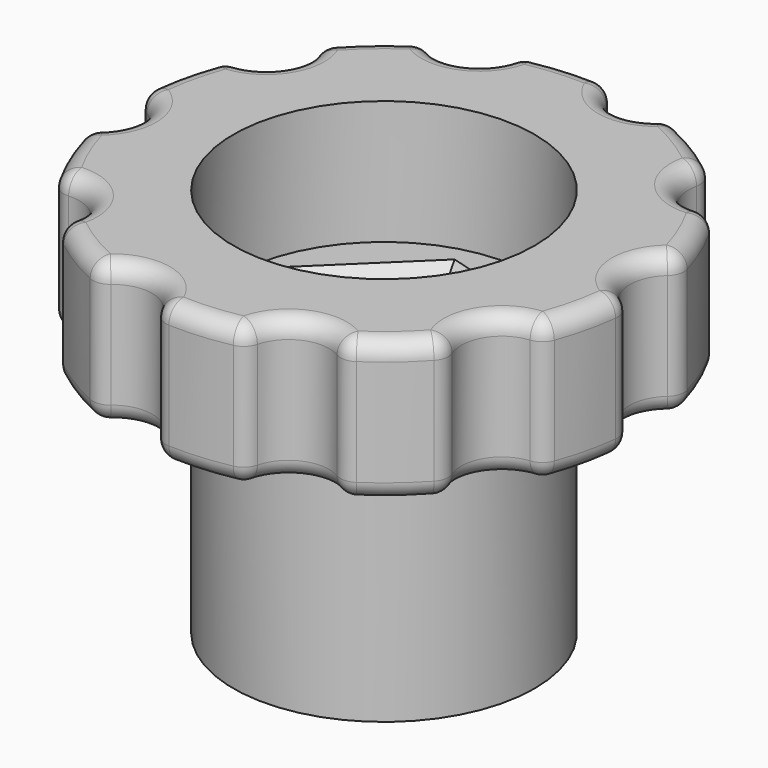
from build123d import *

# Parameters (mm, degrees)
F0_R          = 8.5
F0_R_2        = 2.1
F1_DEPTH      = 5
F2_R          = 8.5
F3_DEPTH      = 10
F4_R          = 8.5
F5_DEPTH      = 7
F5_DEPTH_BACK = 1
F6_SIZE       = 3
F7_R          = 1


with BuildPart() as f1:
    # F0 (on Top) → F1 (new body)
    with BuildSketch(Plane.XY):
        Circle(F0_R)
        Circle(F0_R_2, mode=Mode.SUBTRACT)
    extrude(amount=F1_DEPTH)

    # F2 (on face) → F3 (join)
    with BuildSketch(Plane.XY.offset(5)):
        Circle(F2_R)
        Polygon((2.8988238358, 2.8160528586), (3.8881852318, -1.1024286536), (0.9893613961, -3.9184815122), (-2.8988238358, -2.8160528586), (-3.8881852318, 1.1024286536), (-0.9893613961, 3.9184815122), align=None, mode=Mode.SUBTRACT)
    extrude(amount=F3_DEPTH)

    # F4 (on face) → F5 (join, two sides)
    with BuildSketch(Plane.XY.offset(15)) as f5_sk:
        with BuildLine():
            ThreePointArc((-3.5663232407, 14.0545842536), (-4.9721142928, 11.9370168154), (-7.4654733527, 12.4304749556))
            ThreePointArc((-7.4654733527, 12.4304749556), (-9.4387519636, 11.0072685699), (-11.1462934606, 9.2741653043))
            ThreePointArc((-11.1462934606, 9.2741653043), (-11.0389274013, 6.7347140118), (-13.3461446712, 5.6683703491))
            ThreePointArc((-13.3461446712, 5.6683703491), (-14.1060208777, 3.3571081304), (-14.4687584271, 0.951330426))
            ThreePointArc((-14.4687584271, 0.951330426), (-12.8892454418, -1.0400206398), (-14.1290423441, -3.2588590699))
            ThreePointArc((-14.1290423441, -3.2588590699), (-13.3852692624, -5.575353511), (-12.2646494494, -7.7348803405))
            ThreePointArc((-12.2646494494, -7.7348803405), (-9.8163098129, -8.417502756), (-9.5151260701, -10.9413150887))
            ThreePointArc((-9.5151260701, -10.9413150887), (-7.5517997375, -12.3782196104), (-5.3758612422, -13.4666297159))
            ThreePointArc((-5.3758612422, -13.4666297159), (-2.9938774796, -12.5797849198), (-1.2667550445, -14.4445606253))
            ThreePointArc((-1.2667550445, -14.4445606253), (1.1662006109, -14.4530265389), (3.5663232407, -14.0545842536))
            ThreePointArc((3.5663232407, -14.0545842536), (4.9721142928, -11.9370168154), (7.4654733527, -12.4304749556))
            ThreePointArc((7.4654733527, -12.4304749556), (9.4387519636, -11.0072685699), (11.1462934606, -9.2741653043))
            ThreePointArc((11.1462934606, -9.2741653043), (11.0389274013, -6.7347140118), (13.3461446712, -5.6683703491))
            ThreePointArc((13.3461446712, -5.6683703491), (14.1060208777, -3.3571081304), (14.4687584271, -0.951330426))
            ThreePointArc((14.4687584271, -0.951330426), (12.8892454418, 1.0400206398), (14.1290423441, 3.2588590699))
            ThreePointArc((14.1290423441, 3.2588590699), (13.3852692624, 5.575353511), (12.2646494494, 7.7348803405))
            ThreePointArc((12.2646494494, 7.7348803405), (9.8163098129, 8.417502756), (9.5151260701, 10.9413150887))
            ThreePointArc((9.5151260701, 10.9413150887), (7.5517997375, 12.3782196104), (5.3758612422, 13.4666297159))
            ThreePointArc((5.3758612422, 13.4666297159), (2.9938774796, 12.5797849198), (1.2667550445, 14.4445606253))
            ThreePointArc((1.2667550445, 14.4445606253), (-1.1662006109, 14.4530265389), (-3.5663232407, 14.0545842536))
        make_face()
        Circle(F4_R, mode=Mode.SUBTRACT)
    extrude(amount=F5_DEPTH)
    extrude(f5_sk.sketch, amount=-F5_DEPTH_BACK)

    # F6
    f6_edges = [f1.edges().sort_by_distance(p)[0] for p in [
        (-3.393505, -0.856812, 15),
        (-2.438773, 2.510455, 15),
        (0.954731, 3.367267, 15),
        (-0.954731, -3.367267, 15),
        (2.438773, -2.510455, 15),
        (3.393505, 0.856812, 15),
    ]]
    chamfer(f6_edges, length=F6_SIZE)

    # F7
    f7_edges = [f1.edges().sort_by_distance(p)[0] for p in [
        (-4.972114, 11.937017, 22),
        (-7.465473, 12.430475, 18),
        (-4.972114, 11.937017, 14),
        (-3.566323, 14.054584, 18),
        (2.993877, 12.579785, 22),
        (1.266755, 14.444561, 18),
        (2.993877, 12.579785, 14),
        (5.375861, 13.46663, 18),
        (12.264649, 7.73488, 18),
        (9.81631, 8.417503, 22),
        (9.515126, 10.941315, 18),
        (9.81631, 8.417503, 14),
        (12.889245, 1.040021, 22),
        (14.129042, 3.258859, 18),
        (12.889245, 1.040021, 14),
        (14.468758, -0.95133, 18),
        (11.146293, -9.274165, 18),
        (-11.038927, 6.734714, 22),
        (-13.346145, 5.66837, 18),
        (-11.038927, 6.734714, 14),
        (-11.146293, 9.274165, 18),
        (-4.141177, -4.022933, 13.5),
        (-12.889245, -1.040021, 22),
        (-14.129042, -3.258859, 18),
        (-12.889245, -1.040021, 14),
        (-14.468758, 0.95133, 18),
        (-2.993877, -12.579785, 22),
        (-1.266755, -14.444561, 18),
        (-2.993877, -12.579785, 14),
        (-5.375861, -13.46663, 18),
        (4.972114, -11.937017, 22),
        (7.465473, -12.430475, 18),
        (4.972114, -11.937017, 14),
        (3.566323, -14.054584, 18),
        (-9.81631, -8.417503, 22),
        (-9.515126, -10.941315, 18),
        (-9.81631, -8.417503, 14),
        (-12.264649, -7.73488, 18),
        (11.038927, -6.734714, 22),
        (13.346145, -5.66837, 18),
        (11.038927, -6.734714, 14),
        (13.385269, 5.575354, 22),
        (7.5518, 12.37822, 22),
        (-1.166201, 14.453027, 22),
        (-9.438752, 11.007269, 22),
        (-14.106021, 3.357108, 22),
        (-13.385269, -5.575354, 22),
        (-7.5518, -12.37822, 22),
        (1.166201, -14.453027, 22),
        (9.438752, -11.007269, 22),
        (14.106021, -3.357108, 22),
        (7.5518, 12.37822, 14),
        (-1.166201, 14.453027, 14),
        (-9.438752, 11.007269, 14),
        (-14.106021, 3.357108, 14),
        (-13.385269, -5.575354, 14),
        (-7.5518, -12.37822, 14),
        (1.166201, -14.453027, 14),
        (9.438752, -11.007269, 14),
        (14.106021, -3.357108, 14),
        (13.385269, 5.575354, 14),
        (-8.5, 0, 14),
    ]]
    fillet(f7_edges, radius=F7_R)


solid = f1.part
